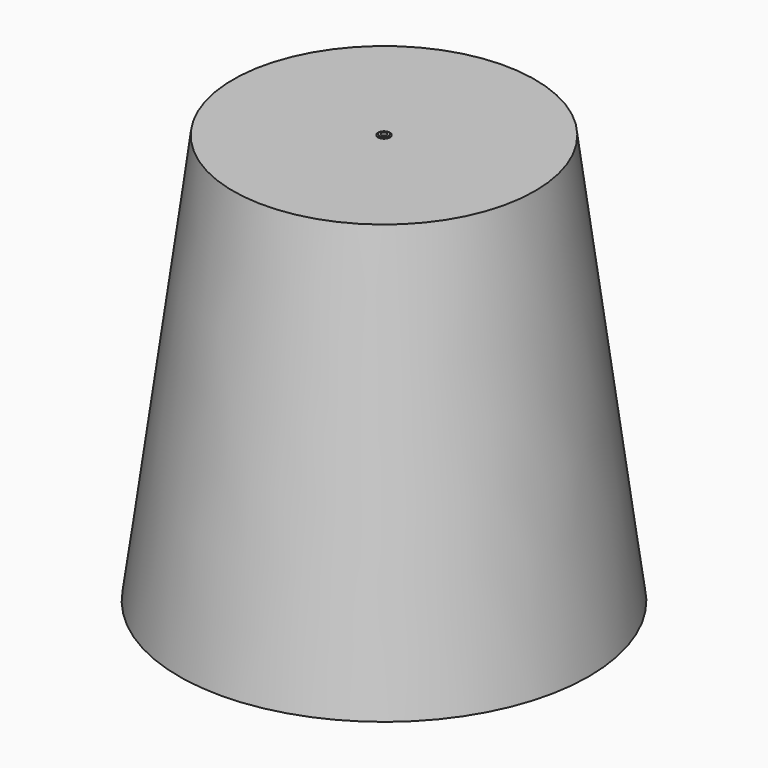
from build123d import *


# Not quite as in the source:
# - a fillet or chamfer that OpenCascade refuses, or shapes differently, is made with other operations: its cross-section is extruded or revolved along the edge and cut away or added


with BuildPart() as f1:
    # F0 (on Front) → F1 (revolve)
    with BuildSketch(Plane.XZ):
        Polygon((5.5, 380), (3.5, 380), (3.5, 379), (5.5, 379), (139.1229595844, 379), (188.991380637, 0), (190, 0), (140, 380), align=None)
    revolve(axis=Axis((0, 0, -10.9773641452), (0, 0, -1)))


with BuildPart() as f2:
    # F0 (on Front) → F2 (revolve)
    with BuildSketch(Plane.XZ):
        Polygon((3.5, 379), (3.5, 380), (5.5, 380), (5.5, 381), (2.5, 381), (2.5, 378), (5.5, 378), (5.5, 379), align=None)
    revolve(axis=Axis((0, 0, -10.9773641452), (0, 0, -1)))

    # F3: chamfer of 1 x 0.5773502692 on 1 edges, made by hand

    # F3_s1 → F3_t2 (revolve, cut)
    with BuildSketch(Plane.XZ):
        Polygon((5.5, 380.4226497308), (4.5, 381), (5.5, 381), align=None)
    revolve(axis=Axis((0, 0, 381), (0, 0, -1)), mode=Mode.SUBTRACT)

    # F4: chamfer of 1 x 0.5773502692 on 1 edges, made by hand

    # F4_s1 → F4_t2 (revolve, cut)
    with BuildSketch(Plane.XZ):
        Polygon((5.5, 378.5773502692), (4.5, 378), (5.5, 378), align=None)
    revolve(axis=Axis((0, 0, 378), (0, 0, -1)), mode=Mode.SUBTRACT)


solid = Compound([f1.part, f2.part])
